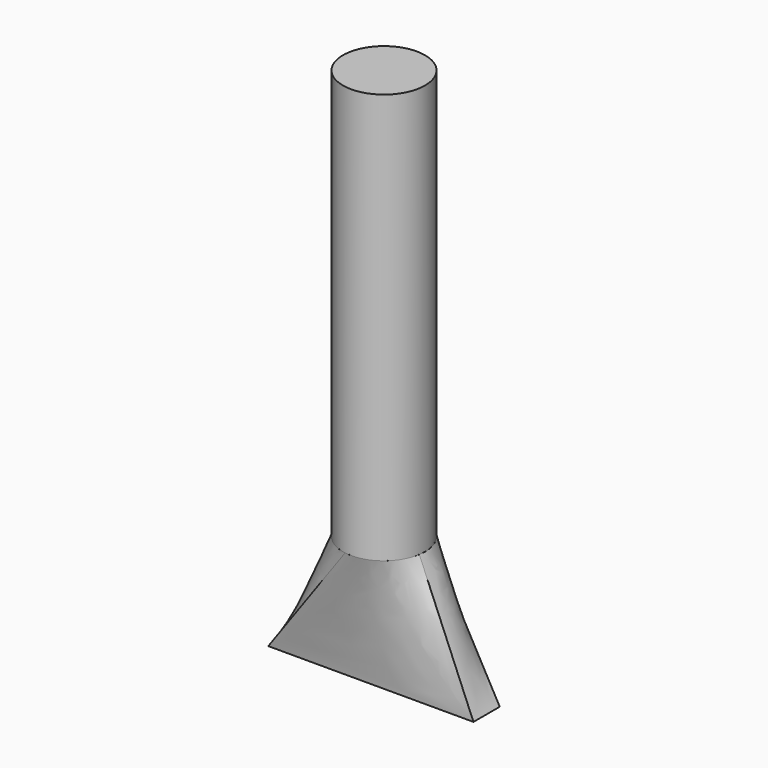
from build123d import *

# Parameters (mm, degrees)
F0_R     = 10
F1_DEPTH = 50
F4_W     = 50
F4_H     = 8
F7_D     = 2.5
F7_DEPTH = 12
F7_TIP   = 0.7510757738


# Not quite as in the source:
# - the arcs of a loft's sections are written as splines that run evenly, so that the points pair up as in the source's solid
# - a feature names something its author has since deleted; it is built from what else it names


with BuildPart() as f1:
    # F0 (on Top) → F1 (new body, symmetric)
    with BuildSketch(Plane.XY):
        Circle(F0_R)
    extrude(amount=F1_DEPTH, both=True)


with BuildPart() as f5:
    # F2 (on face) → F5 section 0
    with BuildSketch(Plane(origin=(0, 0, -50), x_dir=(1, 0, 0), z_dir=(0, 0, -1))):
        with BuildLine():
            add(Edge.make_bspline(
                [(9.8744063192, 1.5799050111), (9.6675972368, 2.8724617757), (9.2038651591, 4.1233892759), (7.832451684, 6.3534379358), (6.9253098794, 7.3316816666), (4.8048863637, 8.8671607642), (3.5924389487, 9.4237919855), (1.0458206508, 10.0309387473), (-0.2873482464, 10.0812154015), (-1.5799050111, 9.8744063192)],
                knots=[0, 0, 0, 0, 0.25, 0.25, 0.5, 0.5, 0.75, 0.75, 1, 1, 1, 1], degree=3))
            add(Edge.make_bspline(
                [(-1.5799050111, 9.8744063192), (-2.8724617757, 9.6675972368), (-4.1233892759, 9.2038651591), (-6.3534379358, 7.832451684), (-7.3316816666, 6.9253098794), (-8.8671607642, 4.8048863637), (-9.4237919855, 3.5924389487), (-10.0309387473, 1.0458206508), (-10.0812154015, -0.2873482464), (-9.8744063192, -1.5799050111)],
                knots=[0, 0, 0, 0, 0.25, 0.25, 0.5, 0.5, 0.75, 0.75, 1, 1, 1, 1], degree=3))
            add(Edge.make_bspline(
                [(-9.8744063192, -1.5799050111), (-9.6675972368, -2.8724617757), (-9.2038651591, -4.1233892759), (-7.832451684, -6.3534379358), (-6.9253098794, -7.3316816666), (-4.8048863637, -8.8671607642), (-3.5924389487, -9.4237919855), (-1.0458206508, -10.0309387473), (0.2873482464, -10.0812154015), (1.5799050111, -9.8744063192)],
                knots=[0, 0, 0, 0, 0.25, 0.25, 0.5, 0.5, 0.75, 0.75, 1, 1, 1, 1], degree=3))
            add(Edge.make_bspline(
                [(1.5799050111, -9.8744063192), (2.8724617757, -9.6675972368), (4.1233892759, -9.2038651591), (6.3534379358, -7.832451684), (7.3316816666, -6.9253098794), (8.8671607642, -4.8048863637), (9.4237919855, -3.5924389487), (10.0309387473, -1.0458206508), (10.0812154015, 0.2873482464), (9.8744063192, 1.5799050111)],
                knots=[0, 0, 0, 0, 0.25, 0.25, 0.5, 0.5, 0.75, 0.75, 1, 1, 1, 1], degree=3))
        make_face()
    # F4 (on offset) → F5 section 1
    with BuildSketch(Plane(origin=(0, 0, -80), x_dir=(1, 0, 0), z_dir=(0, 0, -1))):
        Rectangle(F4_W, F4_H)
    loft(ruled=True)

    # F7
    with Locations(Plane(origin=(0, 0, -80), x_dir=(1, 0, 0), z_dir=(0, 0, -1))):
        with Locations((-17, 0), (-12.5, 0), (-8, 0), (-3.5, 0), (1, 0), (5.5, 0), (10, 0), (14.5, 0)):
            Hole(F7_D / 2, depth=F7_DEPTH)
            with Locations((0, 0, -(F7_DEPTH + F7_TIP / 2))):  # 118° drill point
                Cone(0, F7_D / 2, F7_TIP, mode=Mode.SUBTRACT)


solid = Compound([f1.part, f5.part])
